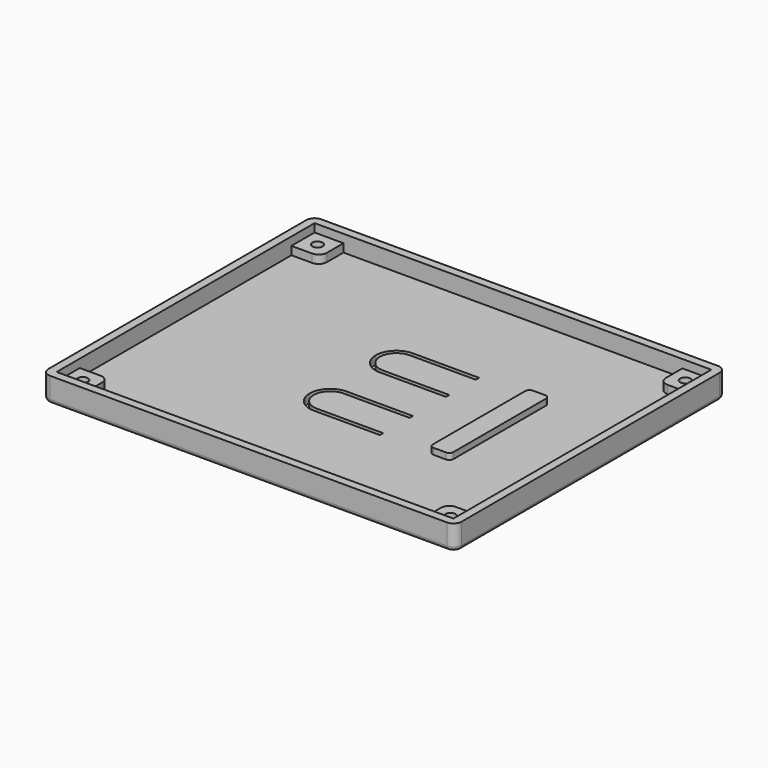
from build123d import *

# Parameters (mm, degrees)
F1_DEPTH  = 2
F2_W      = 96
F2_H      = 78
F3_DEPTH  = 4
F5_DEPTH  = 2
F6_R      = 1.25
F7_DEPTH  = 6
F8_R      = 2.75
F9_DEPTH  = 1.6
F11_R     = 1
F13_DEPTH = 2
F12_R     = 2.5
F14_DEPTH = 1.5
F16_DEPTH = 1.5


# Not quite as in the source:
# - a fillet or chamfer that OpenCascade refuses, or shapes differently, is made with other operations: its cross-section is extruded or revolved along the edge and cut away or added


with BuildPart() as f1:
    # F0 (on Top) → F1 (new body)
    with BuildSketch(Plane.XY):
        with BuildLine():
            ThreePointArc((0, 2), (0.5857864376, 0.5857864376), (2, 0))
            Line((2, 0), (98, 0))
            ThreePointArc((98, 0), (99.4142135624, 0.5857864376), (100, 2))
            Line((100, 2), (100, 80))
            ThreePointArc((100, 80), (99.4142135624, 81.4142135624), (98, 82))
            Line((98, 82), (2, 82))
            ThreePointArc((2, 82), (0.5857864376, 81.4142135624), (0, 80))
            Line((0, 80), (0, 2))
        make_face()
    extrude(amount=F1_DEPTH)

    # F2 (on face) → F3 (join)
    with BuildSketch(Plane.XY.offset(2)):
        with BuildLine():
            ThreePointArc((2, 82), (0.5857864376, 81.4142135624), (0, 80))
            Line((0, 80), (0, 2))
            ThreePointArc((0, 2), (0.5857864376, 0.5857864376), (2, 0))
            Line((2, 0), (98, 0))
            ThreePointArc((98, 0), (99.4142135624, 0.5857864376), (100, 2))
            Line((100, 2), (100, 80))
            ThreePointArc((100, 80), (99.4142135624, 81.4142135624), (98, 82))
            Line((98, 82), (2, 82))
        make_face()
        with Locations((50, 41)):
            Rectangle(F2_W, F2_H, mode=Mode.SUBTRACT)
    extrude(amount=F3_DEPTH)

    # F4 (on face) → F5 (join)
    with BuildSketch(Plane.XY.offset(2)):
        with BuildLine():
            Line((2, 9), (2, 2))
            Line((2, 2), (9, 2))
            Line((9, 2), (9, 7))
            ThreePointArc((9, 7), (8.4142135624, 8.4142135624), (7, 9))
            Line((7, 9), (2, 9))
        make_face()
        with BuildLine():
            Line((9, 80), (2, 80))
            Line((2, 80), (2, 73))
            Line((2, 73), (7, 73))
            ThreePointArc((7, 73), (8.4142135624, 73.5857864376), (9, 75))
            Line((9, 75), (9, 80))
        make_face()
        with BuildLine():
            Line((91, 2), (98, 2))
            Line((98, 2), (98, 9))
            Line((98, 9), (93, 9))
            ThreePointArc((93, 9), (91.5857864376, 8.4142135624), (91, 7))
            Line((91, 7), (91, 2))
        make_face()
        with BuildLine():
            Line((98, 73), (98, 80))
            Line((98, 80), (91, 80))
            Line((91, 80), (91, 75))
            ThreePointArc((91, 75), (91.5857864376, 73.5857864376), (93, 73))
            Line((93, 73), (98, 73))
        make_face()
    extrude(amount=F5_DEPTH)

    # F6 (on face) → F7 (cut)
    with BuildSketch(Plane(origin=(0, 0, 0), x_dir=(1, 0, 0), z_dir=(0, 0, -1))):
        with Locations((94.5, -5.5)):
            Circle(F6_R)
        with Locations((94.5, -76.5)):
            Circle(F6_R)
        with Locations((5.5, -76.5)):
            Circle(F6_R)
        with Locations((5.5, -5.5)):
            Circle(F6_R)
    extrude(amount=-F7_DEPTH, mode=Mode.SUBTRACT)

    # F8 (on face) → F9 (cut)
    with BuildSketch(Plane(origin=(0, 0, 0), x_dir=(1, 0, 0), z_dir=(0, 0, -1))):
        with Locations((5.5, -76.5)):
            Circle(F8_R)
        with Locations((5.5, -5.5)):
            Circle(F8_R)
        with Locations((94.5, -5.5)):
            Circle(F8_R)
        with Locations((94.5, -76.5)):
            Circle(F8_R)
    extrude(amount=-F9_DEPTH, mode=Mode.SUBTRACT)

    # F11
    f11_edges = [f1.edges().sort_by_distance(p)[0] for p in [
        (50, 82, 0),
        (0, 41, 0),
        (0.585786, 81.414214, 0),
        (0.585786, 0.585786, 0),
        (50, 0, 0),
        (99.414214, 81.414214, 0),
        (99.414214, 0.585786, 0),
        (100, 41, 0),
    ]]
    fillet(f11_edges, radius=F11_R)

    # F12 (on face) → F13 (cut)
    with BuildSketch(Plane(origin=(0, 0, 0), x_dir=(1, 0, 0), z_dir=(0, 0, -1))):
        with BuildLine():
            Line((61, -26), (45, -26))
            ThreePointArc((45, -26), (41.4644660941, -27.4644660941), (40, -31))
            ThreePointArc((40, -31), (41.4644660941, -34.5355339059), (45, -36))
            Line((45, -36), (61, -36))
            Line((61, -36), (61, -35))
            Line((61, -35), (45, -35))
            ThreePointArc((45, -35), (42.1715728753, -33.8284271247), (41, -31))
            ThreePointArc((41, -31), (42.1715728753, -28.1715728753), (45, -27))
            Line((45, -27), (61, -27))
            Line((61, -27), (61, -26))
        make_face()
        with BuildLine():
            Line((61, -46), (45, -46))
            ThreePointArc((45, -46), (41.4644660941, -47.4644660941), (40, -51))
            ThreePointArc((40, -51), (41.4644660941, -54.5355339059), (45, -56))
            Line((45, -56), (61, -56))
            Line((61, -56), (61, -55))
            Line((61, -55), (45, -55))
            ThreePointArc((45, -55), (42.1715728753, -53.8284271247), (41, -51))
            ThreePointArc((41, -51), (42.1715728753, -48.1715728753), (45, -47))
            Line((45, -47), (61, -47))
            Line((61, -47), (61, -46))
        make_face()
    extrude(amount=-F13_DEPTH, mode=Mode.SUBTRACT)

    # F12 (on face) → F14 (join)
    with BuildSketch(Plane(origin=(0, 0, 0), x_dir=(1, 0, 0), z_dir=(0, 0, -1))):
        with Locations((45, -51)):
            Circle(F12_R)
        with Locations((45, -31)):
            Circle(F12_R)
    extrude(amount=F14_DEPTH)

    # F15: fillet of radius 2 on 2 edges, made by hand

    # F15_s1 → F15_t2 (revolve, cut)
    with BuildSketch(Plane.XZ.offset(-51)):
        with BuildLine():
            ThreePointArc((47.5, 0), (46.7882531983, -1.0811388301), (45.5635083269, -1.5))
            Line((45.5635083269, -1.5), (47.5, -1.5))
            Line((47.5, -1.5), (47.5, 0))
        make_face()
    revolve(axis=Axis((45, 51, -1.5), (0, 0, -1)), mode=Mode.SUBTRACT)

    # F15_s3 → F15_t4 (revolve, cut)
    with BuildSketch(Plane.XZ.offset(-31)):
        with BuildLine():
            ThreePointArc((47.5, 0), (46.7882531983, -1.0811388301), (45.5635083269, -1.5))
            Line((45.5635083269, -1.5), (47.5, -1.5))
            Line((47.5, -1.5), (47.5, 0))
        make_face()
    revolve(axis=Axis((45, 31, -1.5), (0, 0, -1)), mode=Mode.SUBTRACT)

    # F10 (on face) → F16 (join)
    with BuildSketch(Plane.XY.offset(2)):
        with BuildLine():
            ThreePointArc((73, 27), (73.2928932188, 26.2928932188), (74, 26))
            Line((74, 26), (77, 26))
            ThreePointArc((77, 26), (77.7071067812, 26.2928932188), (78, 27))
            Line((78, 27), (78, 55))
            ThreePointArc((78, 55), (77.7071067812, 55.7071067812), (77, 56))
            Line((77, 56), (74, 56))
            ThreePointArc((74, 56), (73.2928932188, 55.7071067812), (73, 55))
            Line((73, 55), (73, 27))
        make_face()
    extrude(amount=F16_DEPTH)


solid = f1.part
